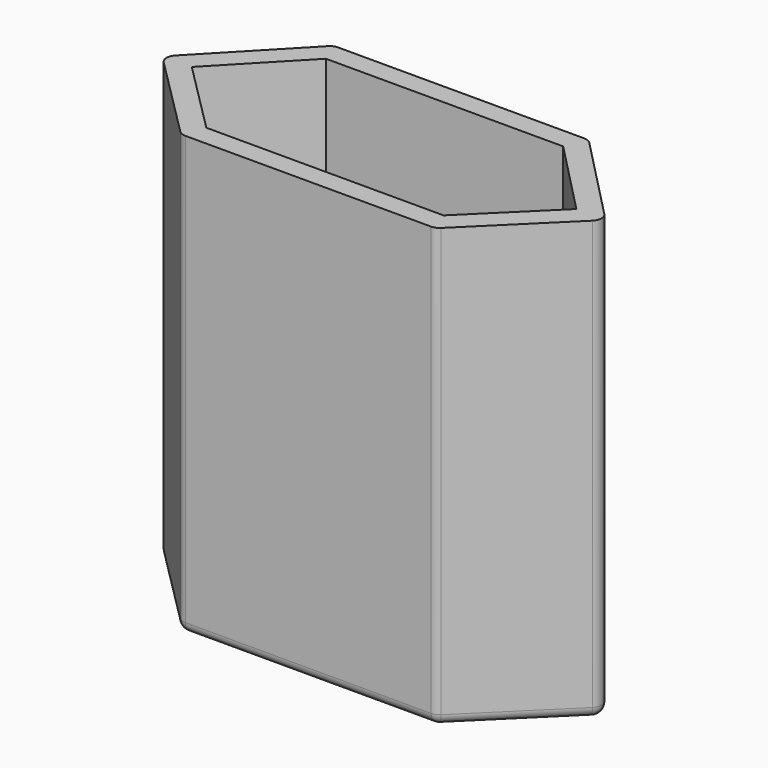
from build123d import *

# Parameters (mm, degrees)
F1_DEPTH     = 42
F2_DEPTH     = 2
F3_R         = 1
F4_T1_DEPTH  = 43.446869231
F4_T3_DEPTH  = 42.0361861213
F4_T5_DEPTH  = 42.0250945478
F4_T7_DEPTH  = 43.4842607953
F4_T9_DEPTH  = 42.0552929075
F4_T11_DEPTH = 42.0664740253
F4_T16_DEPTH = 1
F4_T22_DEPTH = 1
F4_T28_DEPTH = 1
F4_T34_DEPTH = 1
F4_T40_DEPTH = 1
F4_T46_DEPTH = 1


# Not quite as in the source:
# - a fillet or chamfer that OpenCascade refuses, or shapes differently, is made with other operations: its cross-section is extruded or revolved along the edge and cut away or added


with BuildPart() as f1:
    # F0 (on Top) → F1 (new body)
    with BuildSketch(Plane.XY):
        Polygon((-6.2833941388, -9.0027643815), (2.8193882778, -0.0290314764), (-6.2592354511, 9.2972356185), (-30.6566489974, 9.2972356185), (-39.5983849299, -0.0288091293), (-30.6324186742, -9.0027643815), align=None)
        Polygon((-7.1034697771, 7.2972356185), (0, 0), (-7.1034697771, -7.0027643815), (-29.8034697771, -7.0027643815), (-36.8, 0), (-29.8034697771, 7.2972356185), align=None, mode=Mode.SUBTRACT)
    extrude(amount=F1_DEPTH)

    # F0 (on Top) → F2 (join)
    with BuildSketch(Plane.XY):
        Polygon((-7.1034697771, -7.0027643815), (0, 0), (-7.1034697771, 7.2972356185), (-29.8034697771, 7.2972356185), (-36.8, 0), (-29.8034697771, -7.0027643815), align=None)
    extrude(amount=F2_DEPTH)

    # F3
    f3_edges = [f1.edges().sort_by_distance(p)[0] for p in [
        (-1.719924, 4.634102, 0),
        (-18.457942, 9.297236, 0),
        (-35.127517, 4.634213, 0),
        (-35.115402, -4.515787, 0),
        (-18.457906, -9.002764, 0),
        (-1.732003, -4.515898, 0),
    ]]
    fillet(f3_edges, radius=F3_R)

    # F4: fillet of radius 1 on 6 edges, made by hand

    # F4_s2 → F4_t1 (cut)
    with BuildSketch(Plane.XY.offset(1)):
        with BuildLine():
            ThreePointArc((-38.9066140644, -0.7211963873), (-39.1991394765, -0.0246989321), (-38.9210153062, 0.6776733109))
            Line((-38.9210153062, 0.6776733109), (-39.5983849299, -0.0288091293))
            Line((-39.5983849299, -0.0288091293), (-38.9066140644, -0.7211963873))
        make_face()
    extrude(amount=F4_T1_DEPTH, mode=Mode.SUBTRACT)

    # F4_s4 → F4_t3 (cut)
    with BuildSketch(Plane.XY.offset(1)):
        with BuildLine():
            ThreePointArc((-30.2179442256, -9.0027643815), (-30.6008333593, -8.9265586829), (-30.9253658251, -8.7095562041))
            Line((-30.9253658251, -8.7095562041), (-30.6324186742, -9.0027643815))
            Line((-30.6324186742, -9.0027643815), (-30.2179442256, -9.0027643815))
        make_face()
    extrude(amount=F4_T3_DEPTH, mode=Mode.SUBTRACT)

    # F4_s6 → F4_t5 (cut)
    with BuildSketch(Plane.XY.offset(1)):
        with BuildLine():
            ThreePointArc((-5.9913911517, -8.7149011003), (-6.3140487209, -8.9280040042), (-6.693431958, -9.0027643815))
            Line((-6.693431958, -9.0027643815), (-6.2833941388, -9.0027643815))
            Line((-6.2833941388, -9.0027643815), (-5.9913911517, -8.7149011003))
        make_face()
    extrude(amount=F4_T5_DEPTH, mode=Mode.SUBTRACT)

    # F4_s8 → F4_t7 (cut)
    with BuildSketch(Plane.XY.offset(1)):
        with BuildLine():
            ThreePointArc((2.1117349451, -0.726652457), (2.4096411281, -0.0248122758), (2.1262503938, 0.6830135684))
            Line((2.1262503938, 0.6830135684), (2.8193882778, -0.0290314764))
            Line((2.8193882778, -0.0290314764), (2.1117349451, -0.726652457))
        make_face()
    extrude(amount=F4_T7_DEPTH, mode=Mode.SUBTRACT)

    # F4_s10 → F4_t9 (cut)
    with BuildSketch(Plane.XY.offset(1)):
        with BuildLine():
            ThreePointArc((-5.9647963592, 8.9947649251), (-6.2924627239, 9.2185198598), (-6.6813526141, 9.2972356185))
            Line((-6.6813526141, 9.2972356185), (-6.2592354511, 9.2972356185))
            Line((-6.2592354511, 9.2972356185), (-5.9647963592, 8.9947649251))
        make_face()
    extrude(amount=F4_T9_DEPTH, mode=Mode.SUBTRACT)

    # F4_s12 → F4_t11 (cut)
    with BuildSketch(Plane.XY.offset(1)):
        with BuildLine():
            ThreePointArc((-30.2300593872, 9.2972356185), (-30.6224381102, 9.2170393681), (-30.9518822285, 8.9893134941))
            Line((-30.9518822285, 8.9893134941), (-30.6566489974, 9.2972356185))
            Line((-30.6566489974, 9.2972356185), (-30.2300593872, 9.2972356185))
        make_face()
    extrude(amount=F4_T11_DEPTH, mode=Mode.SUBTRACT)


with BuildPart() as f4_tool14:
    # F4_s15 → F4_t16 (new body)
    with BuildSketch(Plane.XY.offset(1)):
        Polygon((-30.2300593872, 8.2972356185), (-30.2300593872, 9.2972356185), (-30.6566489974, 9.2972356185), (-30.9518822285, 8.9893134941), align=None)
    extrude(amount=-F4_T16_DEPTH)

    # F4_s17 → F4_t18 (revolve, cut)
    with BuildSketch(Plane(origin=(-30.2300593872, 8.2972356185, 1), x_dir=(0.3923787229, -0.9198037496, 0), z_dir=(0.9198037496, 0.3923787229, 0))):
        with BuildLine():
            ThreePointArc((0, -1), (1, 0), (0, 1))
            Line((0, 1), (0, -1))
        make_face()
    revolve(axis=Axis((-30.2300593872, 8.2972356185, 1), (0, 0, -1)), mode=Mode.SUBTRACT)


with BuildPart() as f1_1:
    add(f1.part)

    # F4_t13: cut F4_tool14
    add(f4_tool14.part, mode=Mode.SUBTRACT)


with BuildPart() as f4_tool20:
    # F4_s21 → F4_t22 (new body)
    with BuildSketch(Plane.XY.offset(1)):
        Polygon((-6.6813526141, 8.2972356185), (-5.9647963592, 8.9947649251), (-6.2592354511, 9.2972356185), (-6.6813526141, 9.2972356185), align=None)
    extrude(amount=-F4_T22_DEPTH)

    # F4_s23 → F4_t24 (revolve, cut)
    with BuildSketch(Plane(origin=(-6.6813526141, 8.2972356185, 1), x_dir=(-0.3888898902, -0.9212842413, 0), z_dir=(0.9212842413, -0.3888898902, 0))):
        with BuildLine():
            ThreePointArc((0, -1), (1, 0), (0, 1))
            Line((0, 1), (0, -1))
        make_face()
    revolve(axis=Axis((-6.6813526141, 8.2972356185, 1), (0, 0, -1)), mode=Mode.SUBTRACT)


with BuildPart() as f1_2:
    add(f1_1.part)

    # F4_t19: cut F4_tool20
    add(f4_tool20.part, mode=Mode.SUBTRACT)


with BuildPart() as f4_tool26:
    # F4_s27 → F4_t28 (new body)
    with BuildSketch(Plane.XY.offset(1)):
        Polygon((1.4096941389, -0.0145157382), (2.1117349451, -0.726652457), (2.8193882778, -0.0290314764), (2.1262503938, 0.6830135684), align=None)
    extrude(amount=-F4_T28_DEPTH)

    # F4_s29 → F4_t30 (revolve, cut)
    with BuildSketch(Plane(origin=(1.4096941389, -0.0145157382, 1), x_dir=(-0.9999469893, 0.0102965376, 0), z_dir=(-0.0102965376, -0.9999469893, 0))):
        with BuildLine():
            ThreePointArc((0, -1), (1, 0), (0, 1))
            Line((0, 1), (0, -1))
        make_face()
    revolve(axis=Axis((1.4096941389, -0.0145157382, 1), (0, 0, -1)), mode=Mode.SUBTRACT)


with BuildPart() as f1_3:
    add(f1_2.part)

    # F4_t25: cut F4_tool26
    add(f4_tool26.part, mode=Mode.SUBTRACT)


with BuildPart() as f4_tool32:
    # F4_s33 → F4_t34 (new body)
    with BuildSketch(Plane.XY.offset(1)):
        Polygon((-6.693431958, -8.0027643815), (-5.9913911517, -8.7149011003), (-6.2833941388, -9.0027643815), (-6.693431958, -9.0027643815), align=None)
    extrude(amount=-F4_T34_DEPTH)

    # F4_s35 → F4_t36 (revolve, cut)
    with BuildSketch(Plane(origin=(-6.693431958, -8.0027643815, 1), x_dir=(-0.3793832371, 0.9252396227, 0), z_dir=(-0.9252396227, -0.3793832371, 0))):
        with BuildLine():
            ThreePointArc((0, -1), (1, 0), (0, 1))
            Line((0, 1), (0, -1))
        make_face()
    revolve(axis=Axis((-6.693431958, -8.0027643815, 1), (0, 0, -1)), mode=Mode.SUBTRACT)


with BuildPart() as f1_4:
    add(f1_3.part)

    # F4_t31: cut F4_tool32
    add(f4_tool32.part, mode=Mode.SUBTRACT)


with BuildPart() as f4_tool38:
    # F4_s39 → F4_t40 (new body)
    with BuildSketch(Plane.XY.offset(1)):
        Polygon((-30.2179442256, -8.0027643815), (-30.2179442256, -9.0027643815), (-30.6324186742, -9.0027643815), (-30.9253658251, -8.7095562041), align=None)
    extrude(amount=-F4_T40_DEPTH)

    # F4_s41 → F4_t42 (revolve, cut)
    with BuildSketch(Plane(origin=(-30.2179442256, -8.0027643815, 1), x_dir=(0.3828891336, 0.9237943014, 0), z_dir=(-0.9237943014, 0.3828891336, 0))):
        with BuildLine():
            ThreePointArc((0, -1), (1, 0), (0, 1))
            Line((0, 1), (0, -1))
        make_face()
    revolve(axis=Axis((-30.2179442256, -8.0027643815, 1), (0, 0, -1)), mode=Mode.SUBTRACT)


with BuildPart() as f1_5:
    add(f1_4.part)

    # F4_t37: cut F4_tool38
    add(f4_tool38.part, mode=Mode.SUBTRACT)


with BuildPart() as f4_tool44:
    # F4_s45 → F4_t46 (new body)
    with BuildSketch(Plane.XY.offset(1)):
        Polygon((-38.1991924649, -0.0144045646), (-38.9066140644, -0.7211963873), (-39.5983849299, -0.0288091293), (-38.9210153062, 0.6776733109), align=None)
    extrude(amount=-F4_T46_DEPTH)

    # F4_s47 → F4_t48 (revolve, cut)
    with BuildSketch(Plane(origin=(-38.1991924649, -0.0144045646, 1), x_dir=(0.9999470116, 0.0102943674, 0), z_dir=(-0.0102943674, 0.9999470116, 0))):
        with BuildLine():
            ThreePointArc((0, -1), (1, 0), (0, 1))
            Line((0, 1), (0, -1))
        make_face()
    revolve(axis=Axis((-38.1991924649, -0.0144045646, 1), (0, 0, -1)), mode=Mode.SUBTRACT)


with BuildPart() as f1_6:
    add(f1_5.part)

    # F4_t43: cut F4_tool44
    add(f4_tool44.part, mode=Mode.SUBTRACT)


solid = f1_6.part
